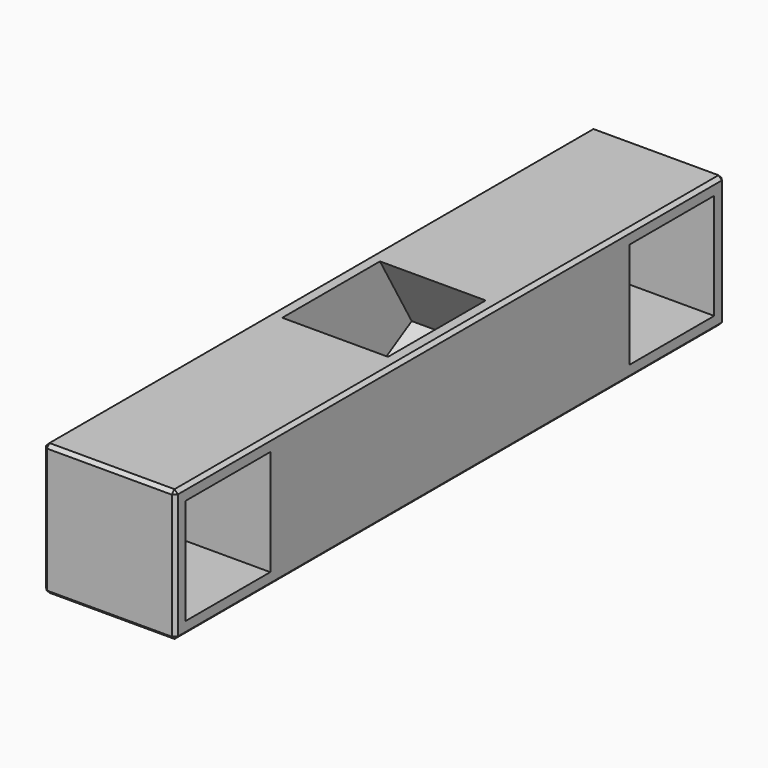
from build123d import *

# Parameters (mm, degrees)
F0_W          = 19.2
F0_H          = 100
F1_DEPTH      = 19.2
F2_W          = 15.4
F2_H          = 15.4
F3_DEPTH      = 18
F5_DEPTH      = 7.7
F5_DEPTH_BACK = 7.7
F6_SIZE       = 0.5


# Not quite as in the source:
# - a pattern or mirror of a feature is missing from the dataset's text; its kind, count and spacing are read off the source's solid


with BuildPart() as f1:
    # F0 (on Top) → F1 (new body)
    with BuildSketch(Plane.XY):
        Rectangle(F0_W, F0_H)
    extrude(amount=F1_DEPTH)

    # F2 (on face) → F3 (cut)
    with BuildSketch(Plane.YZ.offset(9.6)):
        with Locations((-40.4, 9.6)):
            Rectangle(F2_W, F2_H)
    f3 = extrude(amount=-F3_DEPTH, mode=Mode.SUBTRACT)

    # F3_copies: F3 across plane
    add(f3.mirror(Plane.ZX), mode=Mode.SUBTRACT)

    # F4 (on Right) → F5 (cut, two sides)
    with BuildSketch(Plane.YZ) as f5_sk:
        Polygon((1.3316043909, 1.4935935394), (8, 5.3435935394), (14.6683956091, 9.1935935394), (-10.4682390124, 52.7315218353), (-23.8050302307, 45.0315218353), align=None)
    extrude(amount=-F5_DEPTH, mode=Mode.SUBTRACT)
    extrude(f5_sk.sketch, amount=F5_DEPTH_BACK, mode=Mode.SUBTRACT)

    # F6
    f6_edges = [f1.edges().sort_by_distance(p)[0] for p in [
        (-9.6, 50, 9.6),
        (-9.6, -50, 9.6),
        (-9.6, 0, 0),
        (-9.6, 0, 19.2),
        (9.6, -50, 9.6),
        (0, -50, 0),
        (0, -50, 19.2),
        (9.6, 50, 9.6),
        (0, 50, 0),
        (0, 50, 19.2),
        (9.6, 0, 0),
        (9.6, 0, 19.2),
    ]]
    chamfer(f6_edges, length=F6_SIZE)


solid = f1.part
